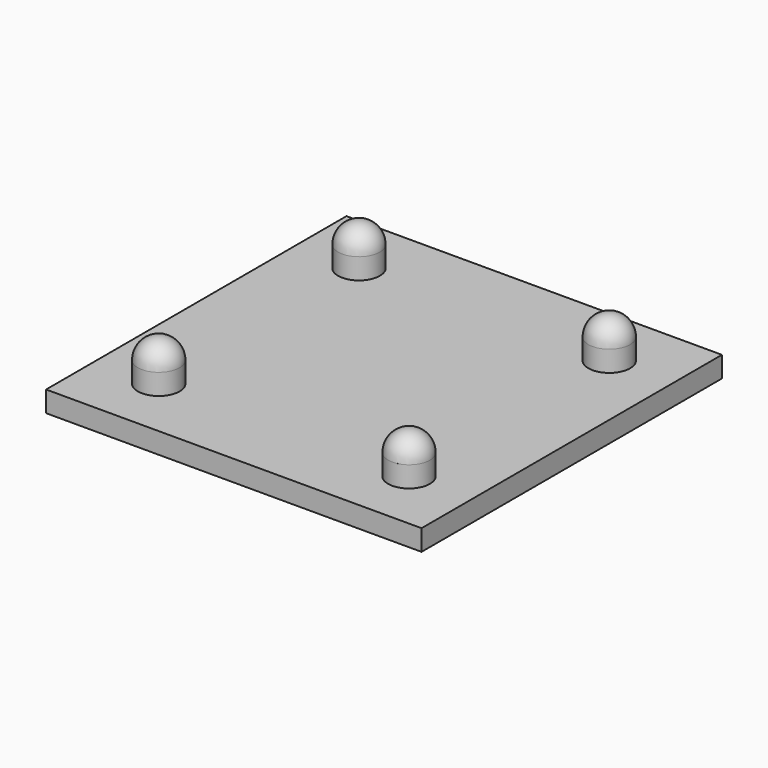
from build123d import *

# Parameters (mm, degrees)
F0_R     = 1.5875
F1_DEPTH = 3.175
F0_W     = 28.575
F0_H     = 28.575
F2_DEPTH = 1.5875


with BuildPart() as f1:
    # F0 (on Top) → F1 (new body)
    with BuildSketch(Plane.XY):
        with Locations((-21.0992920049, 19.05)):
            Circle(F0_R)
    extrude(amount=F1_DEPTH)

    # F7 (on face) → F8 (revolve)
    with BuildSketch(Plane.XY.offset(3.175)):
        with BuildLine():
            Line((-22.6867920049, 19.05), (-21.0992920049, 19.05))
            Line((-21.0992920049, 19.05), (-19.5117920049, 19.05))
            ThreePointArc((-19.5117920049, 19.05), (-21.0992920049, 20.6375), (-22.6867920049, 19.05))
        make_face()
    revolve(axis=Axis((-21.0992920049, 19.05, 3.175), (1, 0, 0)))


with BuildPart() as f1b:
    # F0 (on Top) → F1, piece 2 (new body)
    with BuildSketch(Plane.XY):
        with Locations((-2.0492920049, 19.05)):
            Circle(F0_R)
    extrude(amount=F1_DEPTH)

    # F9 (on face) → F10 (revolve)
    with BuildSketch(Plane.XY.offset(3.175)):
        with BuildLine():
            Line((-0.4617920049, 19.05), (-2.0492920049, 19.05))
            Line((-2.0492920049, 19.05), (-3.6367920049, 19.05))
            ThreePointArc((-3.6367920049, 19.05), (-2.0492920049, 17.4625), (-0.4617920049, 19.05))
        make_face()
    revolve(axis=Axis((-2.0492920049, 19.05, 3.175), (-1, 0, 0)))


with BuildPart() as f1c:
    # F0 (on Top) → F1, piece 3 (new body)
    with BuildSketch(Plane.XY):
        with Locations((-2.0492920049, 0)):
            Circle(F0_R)
    extrude(amount=F1_DEPTH)

    # F5 (on face) → F6 (revolve)
    with BuildSketch(Plane.XY.offset(3.175)):
        with BuildLine():
            Line((-3.6367920049, 0), (-0.4617920049, 0))
            ThreePointArc((-0.4617920049, 0), (-2.0492920049, 1.5875), (-3.6367920049, 0))
        make_face()
    revolve(axis=Axis((-2.0492920049, 0, 3.175), (-1, 0, 0)))


with BuildPart() as f1d:
    # F0 (on Top) → F1, piece 4 (new body)
    with BuildSketch(Plane.XY):
        with Locations((-21.0992920049, 0)):
            Circle(F0_R)
    extrude(amount=F1_DEPTH)

    # F3 (on face) → F4 (revolve)
    with BuildSketch(Plane.XY.offset(3.175)):
        with BuildLine():
            Line((-22.6867920049, 0), (-19.5117920049, 0))
            ThreePointArc((-19.5117920049, 0), (-21.0992920049, 1.5875), (-22.6867920049, 0))
        make_face()
    revolve(axis=Axis((-21.0992920049, 0, 3.175), (-1, 0, 0)))


with BuildPart() as f2:
    # F0 (on Top) → F2 (new body)
    with BuildSketch(Plane.XY):
        with Locations((-11.5742920049, 9.525)):
            Rectangle(F0_W, F0_H)
        with Locations((-21.0992920049, 0)):
            Circle(F0_R, mode=Mode.SUBTRACT)
        with Locations((-2.0492920049, 0)):
            Circle(F0_R, mode=Mode.SUBTRACT)
        with Locations((-21.0992920049, 19.05)):
            Circle(F0_R, mode=Mode.SUBTRACT)
        with Locations((-2.0492920049, 19.05)):
            Circle(F0_R, mode=Mode.SUBTRACT)
    extrude(amount=F2_DEPTH)


solid = Compound([f1.part, f1b.part, f1c.part, f1d.part, f2.part])
